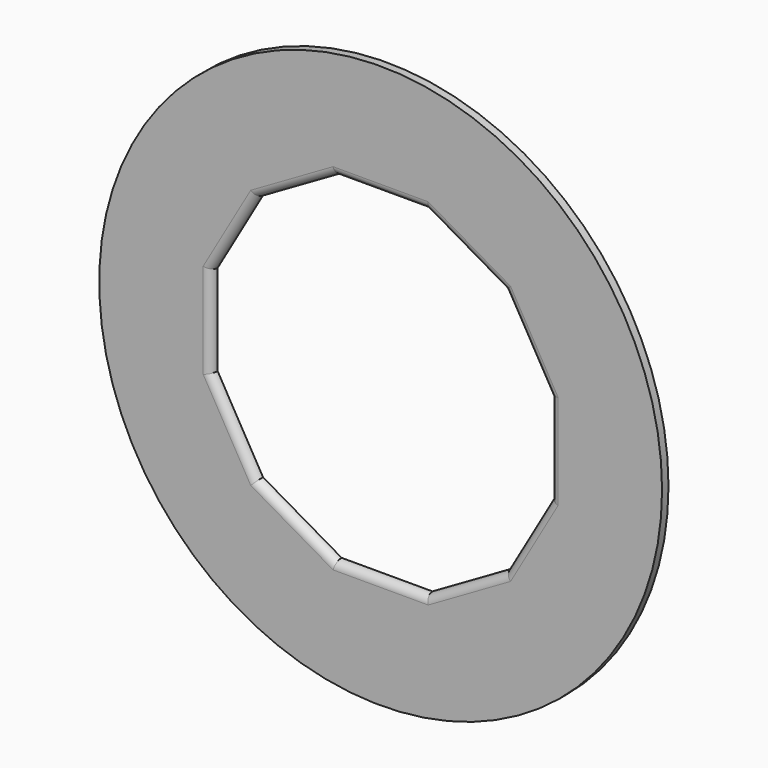
from build123d import *

# Parameters (mm, degrees)
F0_R     = 70
F1_DEPTH = 1
F3_R     = 1.99999


# Not quite as in the source:
# - a fillet or chamfer is up to 0.001 mm smaller than in the source, because OpenCascade refuses the exact size
# - a feature of the source that left no trace in its solid (it failed there, or was rolled back) is left out


with BuildPart() as f1:
    # F0 (on Front) → F1 (new body, symmetric)
    with BuildSketch(Plane.XZ):
        Circle(F0_R)
        Polygon((-30.855941539, 30.855941539), (-11.294058461, 42.15), (11.294058461, 42.15), (30.855941539, 30.855941539), (42.15, 11.294058461), (42.15, -11.294058461), (30.855941539, -30.855941539), (11.294058461, -42.15), (-11.294058461, -42.15), (-30.855941539, -30.855941539), (-42.15, -11.294058461), (-42.15, 11.294058461), align=None, mode=Mode.SUBTRACT)
    extrude(amount=F1_DEPTH, both=True)

    # F3 (radius 2 in the source; OpenCascade refuses exactly that, so slightly less here)
    f3_edges = [f1.edges().sort_by_distance(p)[0] for p in [
        (-21.075, -1, 36.502971),
        (0, -1, 42.15),
        (21.075, -1, 36.502971),
        (36.502971, -1, 21.075),
        (42.15, -1, 0),
        (36.502971, -1, -21.075),
        (21.075, -1, -36.502971),
        (0, -1, -42.15),
        (-21.075, -1, -36.502971),
        (-36.502971, -1, -21.075),
        (-42.15, -1, 0),
        (-36.502971, -1, 21.075),
    ]]
    fillet(f3_edges, radius=F3_R)


solid = f1.part
